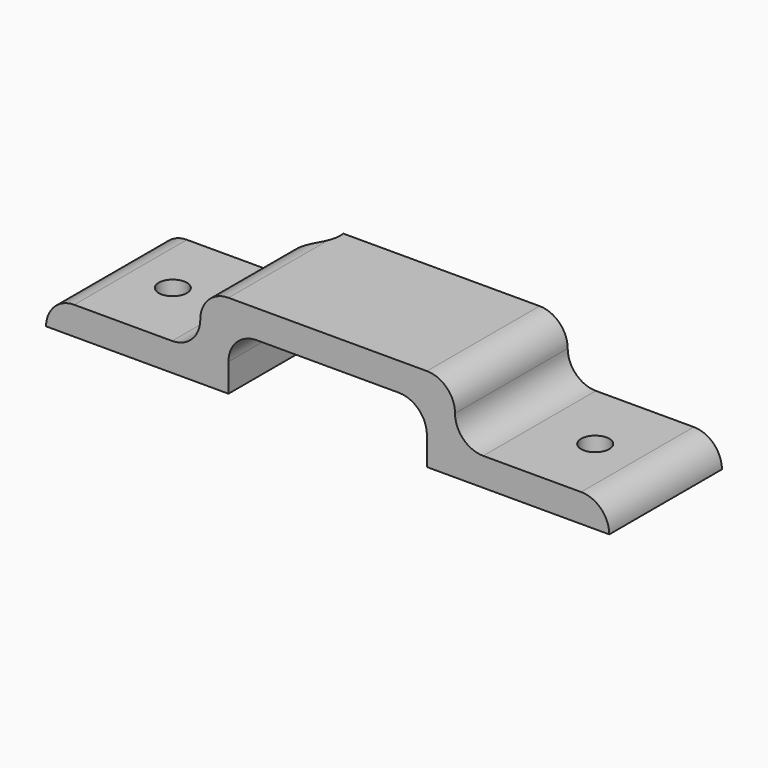
from build123d import *

# Parameters (mm, degrees)
F0_W      = 100
F0_H      = 25
F1_DEPTH  = 5
F2_R      = 2.5
F3_DEPTH  = 25
F4_W      = 45.2307462692
F4_H      = 25
F5_DEPTH  = 10
F6_W      = 35.2307462692
F6_H      = 20
F7_DEPTH  = 78
F8_R      = 4.99999
F9_R      = 5.6856472889
F10_DEPTH = 12.5


# Not quite as in the source:
# - a fillet or chamfer is up to 0.001 mm smaller than in the source, because OpenCascade refuses the exact size


with BuildPart() as f1:
    # F0 (on Top) → F1 (new body)
    with BuildSketch(Plane.XY):
        Rectangle(F0_W, F0_H)
    extrude(amount=F1_DEPTH)

    # F2 (on face) → F3 (cut)
    with BuildSketch(Plane.XY.offset(5)):
        with Locations((-37.5, 0)):
            Circle(F2_R)
        with Locations((37.5, 0)):
            Circle(F2_R)
    extrude(amount=-F3_DEPTH, mode=Mode.SUBTRACT)

    # F4 (on face) → F5 (join)
    with BuildSketch(Plane.XY.offset(5)):
        Rectangle(F4_W, F4_H)
    extrude(amount=F5_DEPTH)

    # F6 (on face) → F7 (cut)
    with BuildSketch(Plane.XZ.offset(12.5)):
        Rectangle(F6_W, F6_H)
    extrude(amount=-F7_DEPTH, mode=Mode.SUBTRACT)

    # F8 (radius 5 in the source; OpenCascade refuses exactly that, so slightly less here)
    f8_edges = [f1.edges().sort_by_distance(p)[0] for p in [
        (22.615373, 0, 5),
        (-22.615373, 0, 5),
        (-22.615373, 0, 15),
        (22.615373, 0, 15),
        (50, 0, 5),
        (-50, 0, 5),
        (-17.615373, 0, 10),
        (17.615373, 0, 10),
    ]]
    fillet(f8_edges, radius=F8_R)

    # F9 (on face) → F10 (cut, symmetric)
    with BuildSketch(Plane.XY.offset(5)):
        with Locations((-22.8596497327, 11.807994917)):
            Circle(F9_R)
    extrude(amount=F10_DEPTH, both=True, mode=Mode.SUBTRACT)


solid = f1.part
